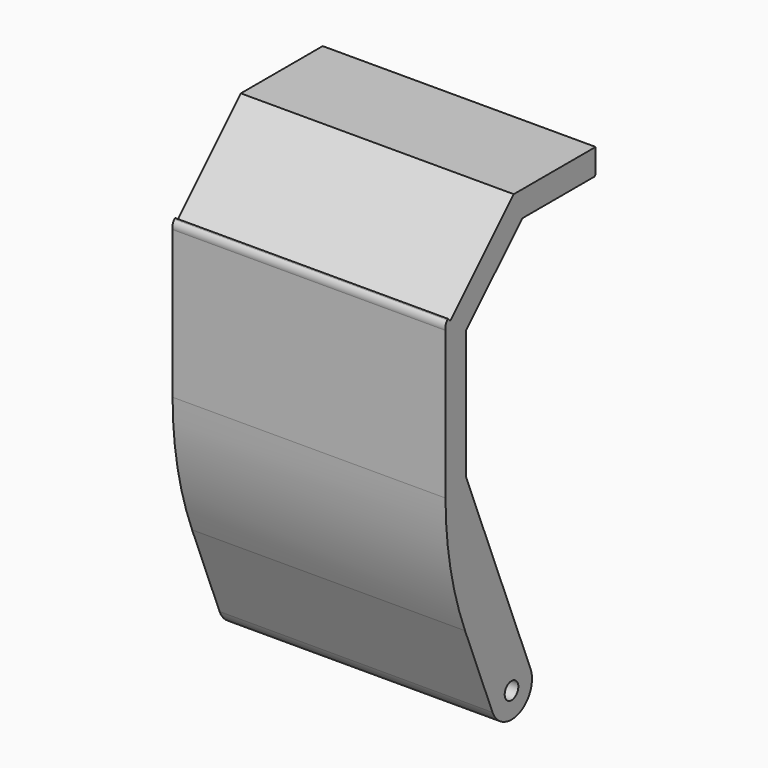
from build123d import *

# Parameters (mm, degrees)
F0_W         = 3
F0_H         = 20
F1_DEPTH     = 10
F2_W         = 3
F2_H         = 20
F3_DEPTH     = 3
F4_DEPTH     = 10
F6_DEPTH     = 25
F7_DEPTH     = 29
F8_R         = 2.99999
F9_R         = 1
F10_DEPTH    = 100
F11_R        = 40
F12_W        = 32
F12_H        = 1
F13_DEPTH    = 0.5
F14_T1_DEPTH = 36.3301270189
F15_SIZE     = 0.2


# Not quite as in the source:
# - a fillet or chamfer that OpenCascade refuses, or shapes differently, is made with other operations: its cross-section is extruded or revolved along the edge and cut away or added
# - a fillet or chamfer is up to 0.001 mm smaller than in the source, because OpenCascade refuses the exact size


with BuildPart() as f1:
    # F0 (on Right) → F1 (new body)
    with BuildSketch(Plane.YZ):
        with Locations((42.2427766025, 31.6474299499)):
            Rectangle(F0_W, F0_H)
    extrude(amount=F1_DEPTH)

    # F2 (on face) → F3 (join)
    with BuildSketch(Plane(origin=(0, 0, 0), x_dir=(0, -1, 0), z_dir=(-1, 0, 0))):
        with Locations((-42.2427766025, 31.6474299499)):
            Rectangle(F2_W, F2_H)
        Polygon((-28.7427766025, 41.6474299499), (-40.7427766025, 41.6474299499), (-40.7427766025, 21.6474299499), (-43.7427766025, 21.6474299499), (-43.7427766025, -18.3525700501), (-28.7427766025, -18.3525700501), (-18.7427766025, 6.6474299499), (-18.7427766025, 31.6474299499), align=None)
    extrude(amount=F3_DEPTH)

    # F4 (cut): a face of the model
    f4_faces = [f1.faces().sort_by_distance(p)[0] for p in [
        (10, 42.2427766025, 31.6474299499),
    ]]
    extrude(f4_faces, amount=-F4_DEPTH, mode=Mode.SUBTRACT)

    # F5 (on face) → F6 (cut)
    with BuildSketch(Plane.YZ):
        Polygon((33.2049743711, -13.3525700501), (26.7427766025, -13.3525700501), (28.7427766025, -18.3525700501), (34.3136367478, -16.124225992), align=None)
        Polygon((41.2427766025, -13.3525700501), (33.2049743711, -13.3525700501), (34.3136367478, -16.124225992), align=None)
        Polygon((34.3136367478, -16.124225992), (28.7427766025, -18.3525700501), (43.7427766025, -18.3525700501), (43.7427766025, -13.3525700501), (41.2427766025, -13.3525700501), align=None)
        Polygon((40.7427766025, 21.6474299499), (43.7427766025, 21.6474299499), (43.7427766025, 41.6474299499), (40.7427766025, 41.6474299499), (40.7427766025, 38.6474299499), align=None)
        Polygon((32.3136367478, -11.124225992), (33.2049743711, -13.3525700501), (41.2427766025, -13.3525700501), (43.7427766025, -12.3525700501), (43.7427766025, 21.6474299499), (40.7427766025, 21.6474299499), (40.7427766025, 38.6474299499), (31.7427766025, 38.6474299499), (29.9854172896, 38.6474299499), (21.7427766025, 30.4047892628), (21.7427766025, 28.6474299499), (21.7427766025, 15.3029243713), (24.3136367478, 8.875774008), align=None)
        Polygon((43.7427766025, -12.3525700501), (41.2427766025, -13.3525700501), (43.7427766025, -13.3525700501), align=None)
        Polygon((32.3136367478, -11.124225992), (26.7427766025, -13.3525700501), (33.2049743711, -13.3525700501), align=None)
    extrude(amount=-F6_DEPTH, mode=Mode.SUBTRACT)

    # F7 (add): a face of the model
    f7_faces = [f1.faces().sort_by_distance(p)[0] for p in [
        (0, 34.7427766025, 41.0550618211),
    ]]
    extrude(f7_faces, amount=F7_DEPTH)

    # F8 (radius 3 in the source; OpenCascade refuses exactly that, so slightly less here)
    f8_edges = [f1.edges().sort_by_distance(p)[0] for p in [
        (13, 26.742777, -13.35257),
        (13, 32.313637, -11.124226),
    ]]
    fillet(f8_edges, radius=F8_R)

    # F9 (on face) → F10 (cut)
    with BuildSketch(Plane.YZ.offset(29)):
        with Locations((28.4140346461, -9.4529679484)):
            Circle(F9_R)
    extrude(amount=-F10_DEPTH, mode=Mode.SUBTRACT)

    # F11
    f11_edges = [f1.edges().sort_by_distance(p)[0] for p in [
        (13, 18.742777, 6.64743),
    ]]
    fillet(f11_edges, radius=F11_R)

    # F12 (on face) → F13 (join)
    with BuildSketch(Plane(origin=(0, -6.4523266737, 6.4523266737), x_dir=(1, 0, 0), z_dir=(0, -0.7071067812, 0.7071067812))):
        with Locations((13, 36.1312567586)):
            Rectangle(F12_W, F12_H)
    extrude(amount=F13_DEPTH)

    # F14: fillet of radius 1 on 1 edges, made by hand

    # F14_s2 → F14_t1 (cut)
    with BuildSketch(Plane.YZ.offset(-5.1650635095)):
        with BuildLine():
            ThreePointArc((18.7427766025, 31.6474299499), (18.7427766025, 32.1650680401), (19.0015956476, 32.6133557762))
            Line((19.0015956476, 32.6133557762), (18.3892232119, 32.0009833405))
            Line((18.3892232119, 32.0009833405), (18.7427766025, 31.6474299499))
        make_face()
    extrude(amount=F14_T1_DEPTH, mode=Mode.SUBTRACT)

    # F15
    f15_edges = [f1.edges().sort_by_distance(p)[0] for p in [
        (13, 40.742777, 38.64743),
    ]]
    chamfer(f15_edges, length=F15_SIZE)


solid = f1.part
